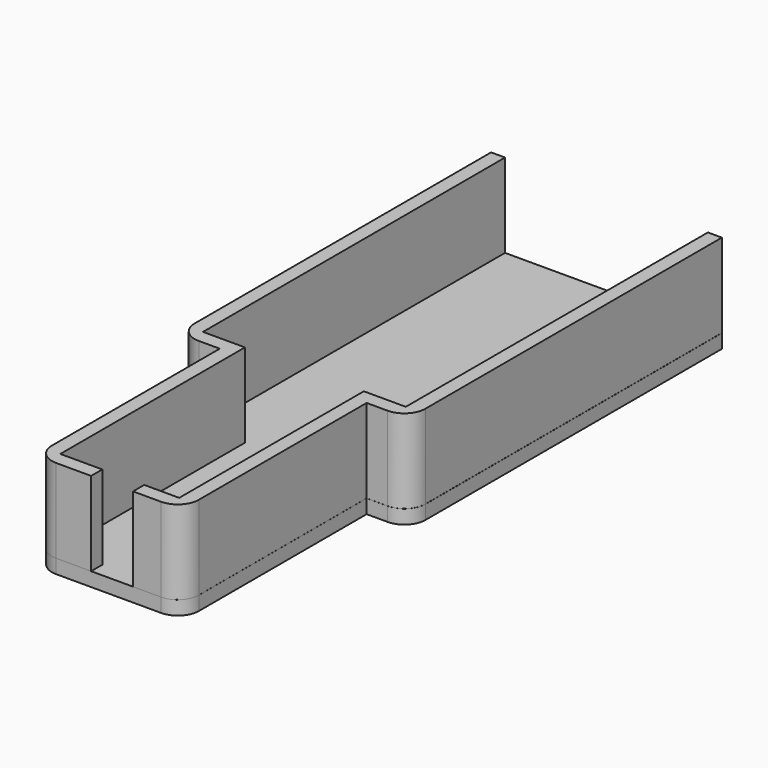
from build123d import *

# Parameters (mm, degrees)
F1_DEPTH = 12
F2_W     = 21.0055973778
F2_H     = 32.9869928685
F3_DEPTH = 2
F4_R     = 3
F4_2_R   = 3
F4_3_R   = 3


with BuildPart() as f1:
    # F0 (on Top) → F1 (new body)
    with BuildSketch(Plane.XY):
        Polygon((-18.4401693158, 45.1313681013), (-20.4401693158, 45.1313681013), (-20.4401693158, -8.8686318987), (-20.4401693158, -10.8686318987), (-14.4401693158, -10.8686318987), (-14.4401693158, -43.8686318987), (-6.4401693158, -43.8686318987), (-6.4401693158, -41.8686318987), (-12.4401693158, -41.8686318987), (-12.4401693158, -8.8686318987), (-18.4401693158, -8.8686318987), align=None)
    extrude(amount=F1_DEPTH)

    # F4
    f4_edges = [f1.edges().sort_by_distance(p)[0] for p in [
        (-20.440169, -10.868632, 6),
        (-14.440169, -43.868632, 6),
    ]]
    fillet(f4_edges, radius=F4_R)


with BuildPart() as f1b:
    # F0 (on Top) → F1, piece 2 (new body)
    with BuildSketch(Plane.XY):
        Polygon((12.5598306842, 45.1313681013), (10.5598306842, 45.1313681013), (10.5598306842, -8.8686318987), (4.5598306842, -8.8686318987), (4.5598306842, -41.8686318987), (-0.4401693158, -41.8686318987), (-0.4401693158, -43.8686318987), (6.5598306842, -43.8686318987), (6.5598306842, -10.8686318987), (12.5598306842, -10.8686318987), (12.5598306842, -8.8686318987), align=None)
    extrude(amount=F1_DEPTH)

    # F4#2
    f4_2_edges = [f1b.edges().sort_by_distance(p)[0] for p in [
        (6.559831, -43.868632, 6),
        (12.559831, -10.868632, 6),
    ]]
    fillet(f4_2_edges, radius=F4_2_R)


with BuildPart() as f1c:
    # F0 (on Top) → F1, piece 3 (new body)
    with BuildSketch(Plane.XY):
        Polygon((-0.4401693158, -43.8701787744), (-0.4401693158, -43.8686318987), (-0.4404736794, -43.8686318987), align=None)
    extrude(amount=F1_DEPTH)


with BuildPart() as f3:
    # F2 (on Top) → F3 (new body)
    with BuildSketch(Plane.XY):
        Polygon((12.5749358821, 45.1223217276), (-20.4250641179, 45.1223217276), (-20.4250641179, -10.8776782724), (-14.4370612154, -10.8776782724), (6.5685361624, -10.8776782724), (12.5749358821, -10.8776782724), align=None)
        with Locations((-3.9342625265, -27.3711747067)):
            Rectangle(F2_W, F2_H)
    extrude(amount=-F3_DEPTH)

    # F4#3
    f4_3_edges = [f3.edges().sort_by_distance(p)[0] for p in [
        (-14.437061, -43.864671, -1),
        (6.568536, -43.864671, -1),
        (12.574936, -10.877678, -1),
        (-20.425064, -10.877678, -1),
    ]]
    fillet(f4_3_edges, radius=F4_3_R)


solid = Compound([f1.part, f1b.part, f1c.part, f3.part])
